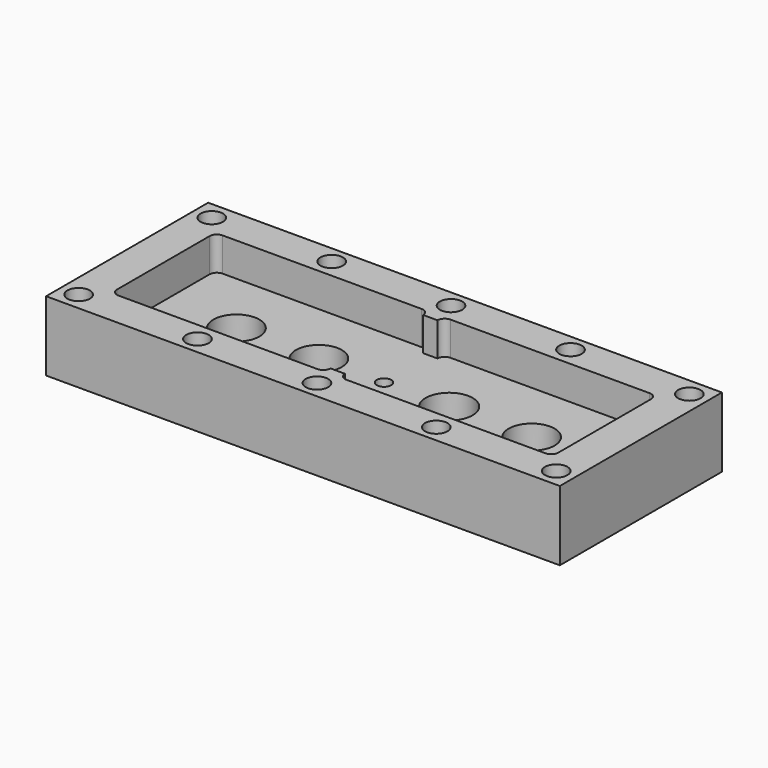
from build123d import *

# Parameters (mm, degrees)
F0_W     = 71
F0_H     = 28
F0_R     = 1.55
F0_W_2   = 2
F0_H_2   = 1
F1_DEPTH = 9.65
F0_R_2   = 3.25
F0_R_3   = 3.175
F2_DEPTH = 5
F3_R     = 0.99999


# Not quite as in the source:
# - a fillet or chamfer is up to 0.001 mm smaller than in the source, because OpenCascade refuses the exact size


with BuildPart() as f1:
    # F0 (on Top) → F1 (new body)
    with BuildSketch(Plane.XY):
        Rectangle(F0_W, F0_H)
        with Locations((-33, -11.5)):
            Circle(F0_R, mode=Mode.SUBTRACT)
        with Locations((-16.5, -11.5939453244)):
            Circle(F0_R, mode=Mode.SUBTRACT)
        with Locations((0, -11.5801189095)):
            Circle(F0_R, mode=Mode.SUBTRACT)
        with Locations((16.5, -11.5939453244)):
            Circle(F0_R, mode=Mode.SUBTRACT)
        with Locations((33, -11.5)):
            Circle(F0_R, mode=Mode.SUBTRACT)
        with Locations((-33, 11.5)):
            Circle(F0_R, mode=Mode.SUBTRACT)
        with Locations((-16.5, 11.5939453244)):
            Circle(F0_R, mode=Mode.SUBTRACT)
        Polygon((-30.5, -9), (-30.5, 9), (-1, 9), (1, 9), (30.5, 9), (30.5, -9), (1, -9), (-1, -9), align=None, mode=Mode.SUBTRACT)
        with Locations((0, 11.5801189095)):
            Circle(F0_R, mode=Mode.SUBTRACT)
        with Locations((16.5, 11.5939453244)):
            Circle(F0_R, mode=Mode.SUBTRACT)
        with Locations((33, 11.5)):
            Circle(F0_R, mode=Mode.SUBTRACT)
        with Locations((0, -8.5)):
            Rectangle(F0_W_2, F0_H_2)
        with Locations((0, 8.5)):
            Rectangle(F0_W_2, F0_H_2)
    extrude(amount=F1_DEPTH)

    # F0 (on Top) → F2 (join)
    with BuildSketch(Plane.XY):
        Polygon((30.5, 9), (1, 9), (1, 8), (1, 0), (1, -8), (1, -9), (30.5, -9), align=None)
        with Locations((9, 0)):
            Circle(F0_R_2, mode=Mode.SUBTRACT)
        with Locations((20.4, 0)):
            Circle(F0_R_3, mode=Mode.SUBTRACT)
        Polygon((-1, 9), (-30.5, 9), (-30.5, -9), (-1, -9), (-1, -8), (-1, -6.4e-09), (-1, 8), align=None)
        with Locations((-20.4, 0)):
            Circle(F0_R_3, mode=Mode.SUBTRACT)
        with Locations((-9, 0)):
            Circle(F0_R_3, mode=Mode.SUBTRACT)
        with BuildLine():
            ThreePointArc((1, 0), (3.2e-09, -1), (-1, -6.4e-09))
            Line((-1, -6.4e-09), (-1, -8))
            Line((-1, -8), (1, -8))
            Line((1, -8), (1, 0))
        make_face()
        with BuildLine():
            Line((1, 8), (-1, 8))
            Line((-1, 8), (-1, -6.4e-09))
            ThreePointArc((-1, -6.4e-09), (-3.2e-09, 1), (1, 0))
            Line((1, 0), (1, 8))
        make_face()
    extrude(amount=F2_DEPTH)

    # F3 (radius 1 in the source; OpenCascade refuses exactly that, so slightly less here)
    f3_edges = [f1.edges().sort_by_distance(p)[0] for p in [
        (-30.5, -9, 7.325),
        (-1, -9, 7.325),
        (-30.5, 9, 7.325),
        (-1, 9, 7.325),
        (1, 9, 7.325),
        (1, -9, 7.325),
        (30.5, -9, 7.325),
        (30.5, 9, 7.325),
    ]]
    fillet(f3_edges, radius=F3_R)


solid = f1.part
